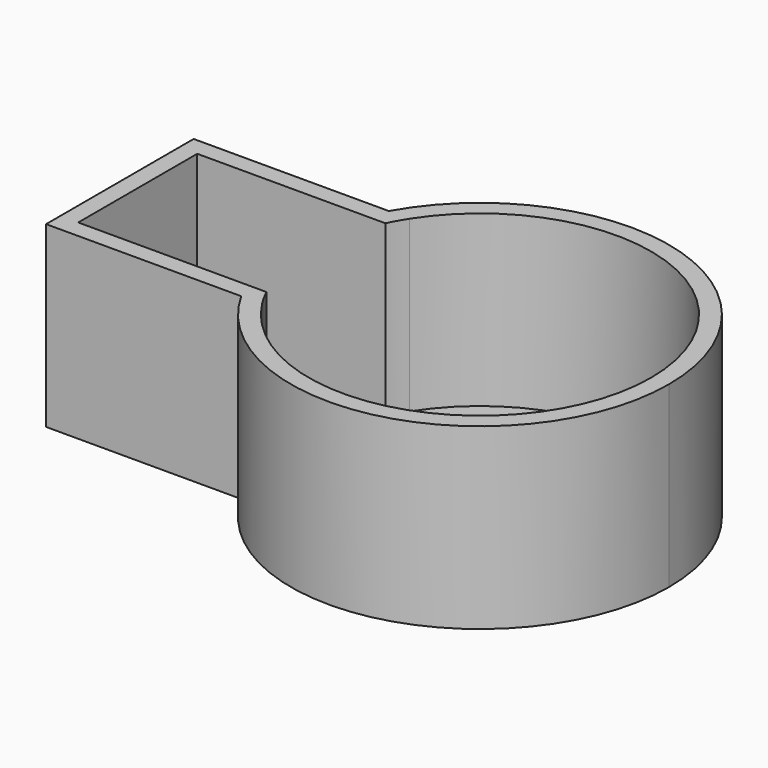
from build123d import *

# Parameters (mm, degrees)
F1_DEPTH = 12
F2_DEPTH = 0.6


with BuildPart() as f1:
    # F0 (on Top) → F1 (new body)
    with BuildSketch(Plane.XY):
        with BuildLine():
            ThreePointArc((-11.6743308159, 5), (-11.3948589306, 5.6077794136), (-11.0837719211, 6.2))
            Line((-11.0837719211, 6.2), (-24.2, 6.2))
            Line((-24.2, 6.2), (-24.2, 0))
            Line((-24.2, 0), (-24.2, -6.2))
            Line((-24.2, -6.2), (-11.0837719211, -6.2))
            ThreePointArc((-11.0837719211, -6.2), (-11.3948589306, -5.6077794136), (-11.6743308159, -5))
            Line((-11.6743308159, -5), (-23, -5))
            Line((-23, -5), (-23, 0))
            Line((-23, 0), (-23, 5))
            Line((-23, 5), (-11.6743308159, 5))
        make_face()
        with BuildLine():
            ThreePointArc((-9.6855562566, 6.2), (3.2300234557, 11.0370715534), (11.5, 0))
            ThreePointArc((11.5, 0), (3.2300234557, -11.0370715534), (-9.6855562566, -6.2))
            Line((-9.6855562566, -6.2), (-11.0837719211, -6.2))
            ThreePointArc((-11.0837719211, -6.2), (3.2035992728, -12.2893023276), (12.7, 0))
            ThreePointArc((12.7, 0), (3.2035992728, 12.2893023276), (-11.0837719211, 6.2))
            Line((-11.0837719211, 6.2), (-9.6855562566, 6.2))
        make_face()
        with BuildLine():
            ThreePointArc((-10.3561575886, 5), (-10.038803388, 5.610029103), (-9.6855562566, 6.2))
            Line((-9.6855562566, 6.2), (-11.0837719211, 6.2))
            ThreePointArc((-11.0837719211, 6.2), (-11.3948589306, 5.6077794136), (-11.6743308159, 5))
            Line((-11.6743308159, 5), (-10.3561575886, 5))
        make_face()
        with BuildLine():
            Line((-11.0837719211, -6.2), (-9.6855562566, -6.2))
            ThreePointArc((-9.6855562566, -6.2), (-10.038803388, -5.610029103), (-10.3561575886, -5))
            Line((-10.3561575886, -5), (-11.6743308159, -5))
            ThreePointArc((-11.6743308159, -5), (-11.3948589306, -5.6077794136), (-11.0837719211, -6.2))
        make_face()
    extrude(amount=F1_DEPTH)

    # F0 (on Top) → F2 (join)
    with BuildSketch(Plane.XY):
        with BuildLine():
            ThreePointArc((-9.6855562566, -6.2), (3.2300234557, -11.0370715534), (11.5, 0))
            ThreePointArc((11.5, 0), (3.2300234557, 11.0370715534), (-9.6855562566, 6.2))
            ThreePointArc((-9.6855562566, 6.2), (-10.038803388, 5.610029103), (-10.3561575886, 5))
            Line((-10.3561575886, 5), (0, 5))
            Line((0, 5), (0, 0))
            Line((0, 0), (-11.5, 0))
            ThreePointArc((-11.5, 0), (-11.2103927734, -2.5645845405), (-10.3561575886, -5))
            ThreePointArc((-10.3561575886, -5), (-10.038803388, -5.610029103), (-9.6855562566, -6.2))
        make_face()
        with BuildLine():
            ThreePointArc((-12.7, 0), (-12.4409405063, 2.5520578596), (-11.6743308159, 5))
            Line((-11.6743308159, 5), (-23, 5))
            Line((-23, 5), (-23, 0))
            Line((-23, 0), (-12.7, 0))
        make_face()
        with BuildLine():
            Line((0, 5), (-10.3561575886, 5))
            ThreePointArc((-10.3561575886, 5), (-11.2103927734, 2.5645845405), (-11.5, 0))
            Line((-11.5, 0), (0, 0))
            Line((0, 0), (0, 5))
        make_face()
        with BuildLine():
            ThreePointArc((-11.5, 0), (-11.2103927734, 2.5645845405), (-10.3561575886, 5))
            Line((-10.3561575886, 5), (-11.6743308159, 5))
            ThreePointArc((-11.6743308159, 5), (-12.4409405063, 2.5520578596), (-12.7, 0))
            Line((-12.7, 0), (-11.5, 0))
        make_face()
        with BuildLine():
            Line((-23, -5), (-11.6743308159, -5))
            ThreePointArc((-11.6743308159, -5), (-12.4409405063, -2.5520578596), (-12.7, 0))
            Line((-12.7, 0), (-23, 0))
            Line((-23, 0), (-23, -5))
        make_face()
        with BuildLine():
            Line((-11.6743308159, -5), (-10.3561575886, -5))
            ThreePointArc((-10.3561575886, -5), (-11.2103927734, -2.5645845405), (-11.5, 0))
            Line((-11.5, 0), (-12.7, 0))
            ThreePointArc((-12.7, 0), (-12.4409405063, -2.5520578596), (-11.6743308159, -5))
        make_face()
    extrude(amount=F2_DEPTH)


solid = f1.part
